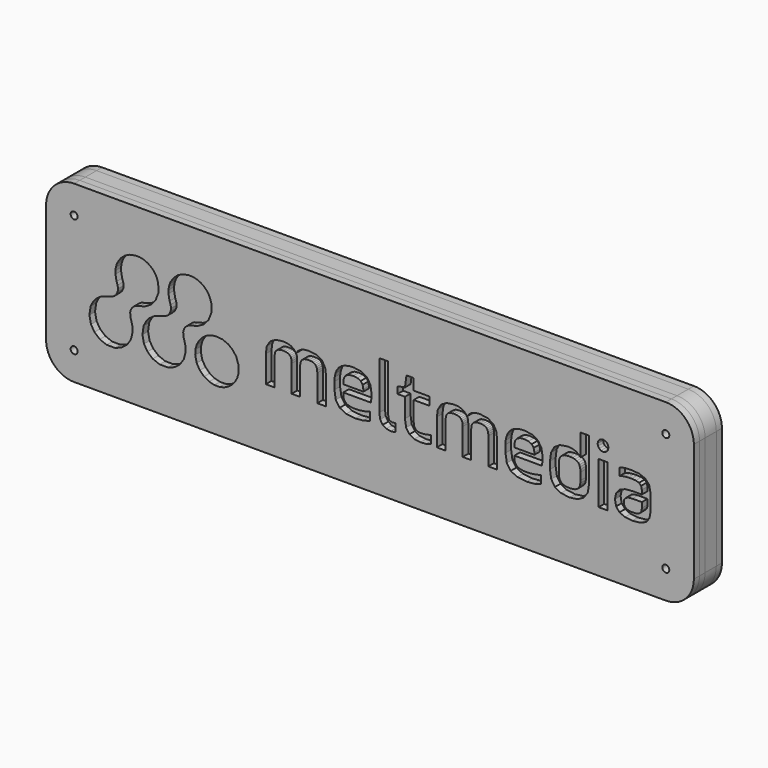
from build123d import *

# Parameters (mm, degrees)
F0_R     = 1.5875
F0_W     = 3.98907
F0_H     = 19.209766
F1_DEPTH = 3.175
F2_DEPTH = 3.175
F3_R     = 1.5875
F4_DEPTH = 6.35
F5_R     = 1.5875
F6_DEPTH = 3.175
F7_SIZE  = 3.17499
F9_DEPTH = 6.35


# Not quite as in the source:
# - a fillet or chamfer is up to 0.001 mm smaller than in the source, because OpenCascade refuses the exact size


with BuildPart() as f1:
    # F0 (on Front) → F1 (new body)
    with BuildSketch(Plane.XZ):
        with BuildLine():
            Line((133.9048122, 39.625524), (-133.9048122, 39.625524))
            ThreePointArc((-133.9048122, 39.625524), (-142.8850683211, 35.9057801211), (-146.6048122, 26.925524))
            Line((-146.6048122, 26.925524), (-146.6048122, -26.747978))
            ThreePointArc((-146.6048122, -26.747978), (-142.8850683211, -35.7282341211), (-133.9048122, -39.447978))
            Line((-133.9048122, -39.447978), (133.9048122, -39.447978))
            ThreePointArc((133.9048122, -39.447978), (142.8850683211, -35.7282341211), (146.6048122, -26.747978))
            Line((146.6048122, -26.747978), (146.6048122, 26.925524))
            ThreePointArc((146.6048122, 26.925524), (142.8850683211, 35.9057801211), (133.9048122, 39.625524))
        make_face()
        with Locations((-133.9048122, -26.747978)):
            Circle(F0_R, mode=Mode.SUBTRACT)
        Polygon((-70.4247258, -19.990562), (-72.7785438, -19.371818), (-75.0564158, -18.125948), (-77.0119618, -16.276828), (-78.4310598, -13.852906), (-79.0983178, -10.884662), (-79.0058618, -8.631428), (-78.4836378, -6.670294), (-77.6553438, -5.001768), (-76.6398518, -3.628898), (-75.4381778, -2.464816), (-73.9469438, -1.46431), (-72.1763098, -0.73787), (-70.0843658, -0.352044), (-66.8240218, -0.596138), (-64.0927598, -1.726184), (-61.9581438, -3.469132), (-60.4864678, -5.559806), (-59.5052658, -8.523732), (-59.4915498, -11.765026), (-60.0620338, -13.778484), (-61.0569518, -15.633446), (-62.4209318, -17.257776), (-64.0968238, -18.578068), (-66.0259538, -19.520662), (-68.1549818, -20.016724), align=None, mode=Mode.SUBTRACT)
        Polygon((-43.1728118, 0.021082), (-43.1728118, -12.099798), (-47.1618818, -12.099798), (-47.1618818, 0.021082), (-46.6907118, 3.205988), (-45.2505318, 5.56514), (-42.8007018, 7.031228), (-39.3003278, 7.534402), (-37.2718838, 7.344156), (-35.6417118, 6.788912), (-34.3889838, 5.901182), (-33.4908398, 4.706874), (-32.5672958, 5.901182), (-31.2983118, 6.788912), (-29.6734738, 7.344156), (-27.6823678, 7.534402), (-24.1075718, 7.042404), (-21.6793318, 5.594096), (-20.2973178, 3.237738), (-19.8591678, 0.021082), (-19.8591678, -12.099798), (-23.8472218, -12.099798), (-23.8472218, 0.021082), (-23.8843058, 0.885444), (-24.0057178, 1.64465), (-24.2343178, 2.295144), (-24.5883938, 2.835402), (-25.0900438, 3.259582), (-25.7595878, 3.566922), (-26.6168378, 3.754374), (-27.6823678, 3.81635), (-28.7626298, 3.754374), (-29.6335958, 3.566922), (-30.3158398, 3.259582), (-30.8284118, 2.835402), (-31.1934098, 2.295144), (-31.4291218, 1.64465), (-31.5558678, 0.885444), (-31.5932058, 0.021082), (-31.5932058, -12.099798), (-35.4651818, -12.099798), (-35.4651818, 0.021082), (-35.5012498, 0.885444), (-35.6183438, 1.64465), (-35.8416098, 2.295144), (-36.1931458, 2.835402), (-36.6920018, 3.259582), (-37.3615458, 3.566922), (-38.2241298, 3.754374), (-39.3003278, 3.81635), (-40.3795738, 3.754374), (-41.2462218, 3.566922), (-41.9213538, 3.259582), (-42.4273218, 2.835402), (-42.7854618, 2.295144), (-43.0143158, 1.64465), (-43.1367438, 0.885444), align=None, mode=Mode.SUBTRACT)
        Polygon((0.6655562, -2.151888), (0.3569462, -3.967988), (-12.0743218, -3.967988), (-12.0743218, -4.81965), (-11.9973598, -5.801106), (-11.7603778, -6.629146), (-11.3539778, -7.31139), (-10.7723178, -7.854188), (-10.0075238, -8.264906), (-9.0524838, -8.548878), (-7.8977998, -8.715248), (-6.5361058, -8.76935), (-4.7555658, -8.679688), (-2.9201618, -8.439912), (-1.2376658, -8.082788), (0.0851662, -7.647432), (0.0851662, -11.402568), (-3.0509718, -12.24026), (-6.5361058, -12.527026), (-10.7377738, -12.063984), (-13.7116058, -10.604754), (-15.4796998, -8.031988), (-16.0638998, -4.238244), (-16.0638998, -0.868934), (-15.9605218, 0.88265), (-15.6310838, 2.48666), (-15.0496778, 3.918204), (-14.1909038, 5.149088), (-13.0296158, 6.152134), (-11.5383818, 6.903212), (-9.6920558, 7.373112), (-7.4649838, 7.534402), (-3.9290498, 7.028688), (-1.3575538, 5.517134), (0.2121662, 3.010154), (0.7437882, -0.481584), align=None, mode=Mode.SUBTRACT)
        with Locations((133.9048122, -26.747978)):
            Circle(F0_R, mode=Mode.SUBTRACT)
        Polygon((12.4778262, 3.390646), (12.4778262, 6.48843), (15.8473902, 7.108444), (16.5060122, 12.142724), (19.7981062, 12.142724), (19.7981062, 7.108444), (26.8468602, 7.108444), (26.8468602, 3.390646), (19.7981062, 3.390646), (19.7981062, -5.40004), (20.0132442, -7.00405), (20.6248762, -8.04291), (21.5786462, -8.602472), (22.8189282, -8.770366), (24.1333782, -8.708644), (25.4135382, -8.537448), (26.5766042, -8.278622), (27.5440902, -7.956296), (27.5440902, -11.674094), (25.3845822, -12.28344), (22.8189282, -12.487148), (20.0295002, -12.130278), (17.8222402, -10.94232), (16.3693602, -8.745728), (15.8473902, -5.361178), (15.8473902, 3.390646), align=None, mode=Mode.SUBTRACT)
        Polygon((34.2438482, 0.021082), (34.2438482, -12.099798), (30.2547782, -12.099798), (30.2547782, 0.021082), (30.7259482, 3.205988), (32.1661282, 5.56514), (34.6162122, 7.031228), (38.1163322, 7.534402), (40.1447762, 7.344156), (41.7749482, 6.788912), (43.0276762, 5.901182), (43.9263282, 4.706874), (44.8496182, 5.901182), (46.1173322, 6.788912), (47.7419162, 7.344156), (49.7348002, 7.534402), (53.3090882, 7.042404), (55.7373282, 5.594096), (57.1195962, 3.237738), (57.5577462, 0.021082), (57.5577462, -12.099798), (53.5684222, -12.099798), (53.5684222, 0.021082), (53.5310842, 0.885444), (53.4099262, 1.64465), (53.1825962, 2.295144), (52.8269962, 2.835402), (52.3253462, 3.259582), (51.6570722, 3.566922), (50.7998222, 3.754374), (49.7348002, 3.81635), (48.6542842, 3.754374), (47.7833182, 3.566922), (47.1013282, 3.259582), (46.5887562, 2.835402), (46.2232502, 2.295144), (45.9875382, 1.64465), (45.8610462, 0.885444), (45.8239622, 0.021082), (45.8239622, -12.099798), (41.9499542, -12.099798), (41.9499542, 0.021082), (41.9154102, 0.885444), (41.7973002, 1.64465), (41.5740342, 2.295144), (41.2240222, 2.835402), (40.7251662, 3.259582), (40.0553682, 3.566922), (39.1927842, 3.754374), (38.1163322, 3.81635), (37.0373402, 3.754374), (36.1704382, 3.566922), (35.4953062, 3.259582), (34.9898462, 2.835402), (34.6311982, 2.295144), (34.4025982, 1.64465), (34.2799162, 0.885444), align=None, mode=Mode.SUBTRACT)
        Polygon((78.0822162, -2.151888), (77.7736062, -3.967988), (65.3423382, -3.967988), (65.3423382, -4.81965), (65.4195542, -5.801106), (65.6562822, -6.629146), (66.0631902, -7.31139), (66.6445962, -7.854188), (67.4093902, -8.264906), (68.3641762, -8.548878), (69.5193682, -8.715248), (70.8805542, -8.76935), (72.6610942, -8.679688), (74.4964982, -8.439912), (76.1792482, -8.082788), (77.5033502, -7.647432), (77.5033502, -11.402568), (74.3656882, -12.24026), (70.8805542, -12.527026), (66.6791402, -12.063984), (63.7050542, -10.604754), (61.9369602, -8.031988), (61.3527602, -4.238244), (61.3527602, -0.868934), (61.4561382, 0.88265), (61.7855762, 2.48666), (62.3669822, 3.918204), (63.2257562, 5.149088), (64.3872982, 6.152134), (65.8782782, 6.903212), (67.7251122, 7.373112), (69.9516762, 7.534402), (73.4881182, 7.028688), (76.0593602, 5.517134), (77.6288262, 3.010154), (78.1609562, -0.481584), align=None, mode=Mode.SUBTRACT)
        with Locations((105.4838632, -2.496439)):
            Rectangle(F0_W, F0_H, mode=Mode.SUBTRACT)
        Polygon((126.9960122, 1.182878), (126.9960122, -6.330188), (126.5134122, -9.09574), (125.0198922, -11.026394), (122.4544922, -12.15771), (118.7486322, -12.527026), (115.3958322, -12.171426), (112.9294922, -11.084306), (111.4054922, -9.22655), (110.8873322, -6.563106), (111.4385122, -3.817874), (113.0209322, -2.011172), (115.5101322, -1.017778), (118.7867322, -0.714756), (123.0463122, -0.714756), (123.0463122, 1.182878), (122.7186522, 2.657602), (121.7915522, 3.556), (120.3488322, 4.005072), (118.4768522, 4.126484), (116.8258522, 4.0767), (115.3323322, 3.933444), (114.0369322, 3.70205), (112.9777522, 3.390646), (112.9777522, 6.87578), (115.3475722, 7.380224), (118.2431722, 7.534402), (121.8169522, 7.222744), (124.5804722, 6.174232), (126.3635522, 4.21894), align=None, mode=Mode.SUBTRACT)
        Polygon((-108.2463418, -2.313178), (-108.5386958, -3.510534), (-108.3690238, -5.424678), (-107.8950598, -7.140194), (-107.5064398, -8.887968), (-107.4276998, -10.945368), (-108.2450718, -14.208506), (-110.0060538, -16.862298), (-112.4962698, -18.78076), (-115.5018518, -19.839178), (-119.1907954, -19.839178), (-122.2982822, -18.631916), (-124.7002078, -16.56461), (-126.2711724, -13.98651), (-126.9960122, -10.529062), (-126.44755, -6.846824), (-125.4043974, -4.764532), (-123.9381316, -2.996438), (-122.07367, -1.617218), (-119.8343552, -0.702056), (-118.1572694, -0.294132), (-116.5574758, 0.236474), (-115.5859258, 0.853694), (-114.7797298, 1.738376), (-114.2338838, 2.865628), (-114.0383038, 4.211828), (-114.2724918, 5.567934), (-114.6847338, 6.848094), (-115.2097518, 9.59866), (-115.2122918, 11.056874), (-115.0098538, 12.452604), (-114.6296158, 13.753338), (-114.0974858, 14.924532), (-112.8008158, 16.7767), (-110.9956378, 18.378424), (-108.7535798, 19.476466), (-105.9628818, 20.016724), (-103.9829518, 19.937984), (-102.1417058, 19.472402), (-100.5143278, 18.722594), (-99.1734618, 17.793716), (-98.0434158, 16.705072), (-97.0871058, 15.432024), (-96.3403458, 13.935456), (-95.8371718, 12.17295), (-95.8125338, 8.277352), (-97.0952338, 5.019294), (-99.3151938, 2.543302), (-102.1003038, 0.994156), (-104.1013158, 0.518922), (-106.0802298, -0.059944), (-106.9402738, -0.589026), (-107.6883038, -1.340104), align=None, mode=Mode.SUBTRACT)
        Polygon((-84.2476598, -2.313178), (-84.5412838, -3.510534), (-84.3718658, -5.424678), (-83.8963778, -7.140194), (-83.5092818, -8.887968), (-83.4292718, -10.945368), (-84.2476598, -14.208506), (-86.0091498, -16.862298), (-88.5003818, -18.78076), (-91.5062178, -19.839178), (-95.1950598, -19.839178), (-98.3024958, -18.631916), (-100.7045738, -16.56461), (-102.2753098, -13.98651), (-102.9989558, -10.529062), (-102.4503158, -6.846824), (-101.4071378, -4.764532), (-99.9410498, -2.996438), (-98.0766898, -1.617218), (-95.8371718, -0.702056), (-94.1600098, -0.294132), (-92.5587938, 0.236474), (-91.5887678, 0.853694), (-90.7840958, 1.738376), (-90.2382498, 2.865628), (-90.0439398, 4.211828), (-90.2753338, 5.567934), (-90.6860518, 6.848094), (-91.2125938, 9.59866), (-91.2151338, 11.056874), (-91.0126958, 12.452604), (-90.6322038, 13.753338), (-90.1003278, 14.924532), (-88.8049278, 16.7767), (-86.9997498, 18.378424), (-84.7564218, 19.476466), (-81.9631838, 20.016724), (-79.9855398, 19.937984), (-78.1448018, 19.472402), (-76.5169158, 18.722594), (-75.1750338, 17.793716), (-74.0460038, 16.705072), (-73.0902018, 15.432024), (-72.3429338, 13.935456), (-71.8402678, 12.17295), (-71.8151218, 8.277352), (-73.0980758, 5.019294), (-75.3167658, 2.543302), (-78.1031458, 0.994156), (-80.1054278, 0.518922), (-82.0818018, -0.059944), (-82.9428618, -0.589026), (-83.6896218, -1.340104), align=None, mode=Mode.SUBTRACT)
        with Locations((-133.9048122, 26.925524)):
            Circle(F0_R, mode=Mode.SUBTRACT)
        Polygon((4.2289222, -6.678676), (4.2289222, 15.00886), (8.2200242, 15.00886), (8.2200242, -5.904484), (8.3399122, -7.24789), (8.6927182, -8.09117), (9.2644722, -8.52805), (10.0389182, -8.653272), (10.7884722, -8.609076), (11.5105942, -8.421878), (11.5105942, -12.061444), (10.5763822, -12.321794), (9.3802962, -12.409932), (7.3655682, -12.097004), (5.7295542, -11.098022), (4.6299882, -9.3218), align=None, mode=Mode.SUBTRACT)
        Polygon((99.1911402, 15.00886), (99.1911402, -4.238244), (98.5723962, -7.917688), (96.8083662, -10.501376), (94.0260502, -12.025376), (90.3605762, -12.525756), (86.4911402, -12.025376), (83.7184762, -10.501376), (82.0481722, -7.917688), (81.4914042, -4.238244), (81.4914042, -0.907288), (81.9656222, 2.65049), (83.4317102, 5.303266), (85.9524062, 6.962394), (89.5858762, 7.534402), (91.5746962, 7.359396), (93.1525442, 6.856222), (94.3610762, 6.063996), (95.2401702, 5.016754), (95.2401702, 15.00886), align=None, mode=Mode.SUBTRACT)
        Polygon((104.5434282, 15.28318), (105.5035482, 15.473172), (106.4560482, 15.277338), (107.2304942, 14.748256), (107.7514482, 13.971016), (107.9432182, 13.03401), (107.7514482, 12.082018), (107.2304942, 11.306302), (106.4560482, 10.785094), (105.5035482, 10.593578), (104.5434282, 10.785094), (103.7550122, 11.306302), (103.2205962, 12.082018), (103.0247622, 13.03401), (103.2205962, 13.98778), (103.7550122, 14.762226), align=None, mode=Mode.SUBTRACT)
        with Locations((133.9048122, 26.925524)):
            Circle(F0_R, mode=Mode.SUBTRACT)
    extrude(amount=F1_DEPTH)


with BuildPart() as f1b:
    # F0 (on Front) → F1, piece 2 (new body)
    with BuildSketch(Plane.XZ):
        Polygon((-12.0743218, 0.254254), (-12.0743218, -0.714756), (-3.0126178, -0.714756), (-3.0126178, 0.254254), (-3.3184338, 1.964182), (-4.2087038, 3.159252), (-5.6432958, 3.860546), (-7.5820778, 4.087876), (-9.5099378, 3.860546), (-10.9183678, 3.159252), (-11.7822218, 1.964182), align=None)
    extrude(amount=F1_DEPTH)


with BuildPart() as f1c:
    # F0 (on Front) → F1, piece 3 (new body)
    with BuildSketch(Plane.XZ):
        Polygon((65.3423382, 0.254254), (65.3423382, -0.714756), (74.4042962, -0.714756), (74.4042962, 0.254254), (74.0982262, 1.964182), (73.2082102, 3.159252), (71.7736182, 3.860546), (69.8345822, 4.087876), (67.9067222, 3.860546), (66.4985462, 3.159252), (65.6344382, 1.964182), align=None)
    extrude(amount=F1_DEPTH)


with BuildPart() as f1d:
    # F0 (on Front) → F1, piece 4 (new body)
    with BuildSketch(Plane.XZ):
        Polygon((85.4809822, -0.830326), (85.4809822, -4.161028), (85.5236542, -5.226304), (85.6697042, -6.154928), (85.9496122, -6.946138), (86.3905562, -7.597648), (87.0186982, -8.107934), (87.8647722, -8.474456), (88.9562102, -8.696198), (90.3219682, -8.770366), (91.6778202, -8.696198), (92.7723062, -8.474456), (93.6305722, -8.107934), (94.2754782, -7.597648), (94.7344562, -6.946138), (95.0321442, -6.154928), (95.1919102, -5.226304), (95.2401702, -4.161028), (95.2401702, -0.830326), (95.1919102, 0.237744), (95.0321442, 1.170432), (94.7344562, 1.9685), (94.2754782, 2.625852), (93.6305722, 3.144012), (92.7723062, 3.516122), (91.6778202, 3.741928), (90.3219682, 3.81635), (88.9785622, 3.741928), (87.8980462, 3.516122), (87.0534962, 3.144012), (86.4195122, 2.625852), (85.9699322, 1.9685), (85.6806262, 1.170432), (85.5264482, 0.237744), align=None)
    extrude(amount=F1_DEPTH)


with BuildPart() as f1e:
    # F0 (on Front) → F1, piece 5 (new body)
    with BuildSketch(Plane.XZ):
        Polygon((123.0463122, -6.137148), (123.0463122, -3.73507), (118.7867322, -3.73507), (117.0646122, -3.886962), (115.8428722, -4.369054), (115.1138922, -5.22224), (114.8751322, -6.48589), (115.1875522, -7.866634), (116.0308322, -8.678418), (117.2424122, -9.06145), (118.6698922, -9.157716), (119.5817522, -9.135872), (120.4148722, -9.055862), (121.1590922, -8.896096), (121.8017122, -8.634222), (122.3249522, -8.249666), (122.7161122, -7.71906), (122.9599522, -7.021576), align=None)
    extrude(amount=F1_DEPTH)


with BuildPart() as f2:
    # F0 (on Front) → F2 (new body)
    with BuildSketch(Plane.XZ):
        with BuildLine():
            Line((133.9048122, 39.625524), (-133.9048122, 39.625524))
            ThreePointArc((-133.9048122, 39.625524), (-142.8850683211, 35.9057801211), (-146.6048122, 26.925524))
            Line((-146.6048122, 26.925524), (-146.6048122, -26.747978))
            ThreePointArc((-146.6048122, -26.747978), (-142.8850683211, -35.7282341211), (-133.9048122, -39.447978))
            Line((-133.9048122, -39.447978), (133.9048122, -39.447978))
            ThreePointArc((133.9048122, -39.447978), (142.8850683211, -35.7282341211), (146.6048122, -26.747978))
            Line((146.6048122, -26.747978), (146.6048122, 26.925524))
            ThreePointArc((146.6048122, 26.925524), (142.8850683211, 35.9057801211), (133.9048122, 39.625524))
        make_face()
        with Locations((-133.9048122, -26.747978)):
            Circle(F0_R, mode=Mode.SUBTRACT)
        Polygon((-70.4247258, -19.990562), (-72.7785438, -19.371818), (-75.0564158, -18.125948), (-77.0119618, -16.276828), (-78.4310598, -13.852906), (-79.0983178, -10.884662), (-79.0058618, -8.631428), (-78.4836378, -6.670294), (-77.6553438, -5.001768), (-76.6398518, -3.628898), (-75.4381778, -2.464816), (-73.9469438, -1.46431), (-72.1763098, -0.73787), (-70.0843658, -0.352044), (-66.8240218, -0.596138), (-64.0927598, -1.726184), (-61.9581438, -3.469132), (-60.4864678, -5.559806), (-59.5052658, -8.523732), (-59.4915498, -11.765026), (-60.0620338, -13.778484), (-61.0569518, -15.633446), (-62.4209318, -17.257776), (-64.0968238, -18.578068), (-66.0259538, -19.520662), (-68.1549818, -20.016724), align=None, mode=Mode.SUBTRACT)
        Polygon((-43.1728118, 0.021082), (-43.1728118, -12.099798), (-47.1618818, -12.099798), (-47.1618818, 0.021082), (-46.6907118, 3.205988), (-45.2505318, 5.56514), (-42.8007018, 7.031228), (-39.3003278, 7.534402), (-37.2718838, 7.344156), (-35.6417118, 6.788912), (-34.3889838, 5.901182), (-33.4908398, 4.706874), (-32.5672958, 5.901182), (-31.2983118, 6.788912), (-29.6734738, 7.344156), (-27.6823678, 7.534402), (-24.1075718, 7.042404), (-21.6793318, 5.594096), (-20.2973178, 3.237738), (-19.8591678, 0.021082), (-19.8591678, -12.099798), (-23.8472218, -12.099798), (-23.8472218, 0.021082), (-23.8843058, 0.885444), (-24.0057178, 1.64465), (-24.2343178, 2.295144), (-24.5883938, 2.835402), (-25.0900438, 3.259582), (-25.7595878, 3.566922), (-26.6168378, 3.754374), (-27.6823678, 3.81635), (-28.7626298, 3.754374), (-29.6335958, 3.566922), (-30.3158398, 3.259582), (-30.8284118, 2.835402), (-31.1934098, 2.295144), (-31.4291218, 1.64465), (-31.5558678, 0.885444), (-31.5932058, 0.021082), (-31.5932058, -12.099798), (-35.4651818, -12.099798), (-35.4651818, 0.021082), (-35.5012498, 0.885444), (-35.6183438, 1.64465), (-35.8416098, 2.295144), (-36.1931458, 2.835402), (-36.6920018, 3.259582), (-37.3615458, 3.566922), (-38.2241298, 3.754374), (-39.3003278, 3.81635), (-40.3795738, 3.754374), (-41.2462218, 3.566922), (-41.9213538, 3.259582), (-42.4273218, 2.835402), (-42.7854618, 2.295144), (-43.0143158, 1.64465), (-43.1367438, 0.885444), align=None, mode=Mode.SUBTRACT)
        Polygon((0.6655562, -2.151888), (0.3569462, -3.967988), (-12.0743218, -3.967988), (-12.0743218, -4.81965), (-11.9973598, -5.801106), (-11.7603778, -6.629146), (-11.3539778, -7.31139), (-10.7723178, -7.854188), (-10.0075238, -8.264906), (-9.0524838, -8.548878), (-7.8977998, -8.715248), (-6.5361058, -8.76935), (-4.7555658, -8.679688), (-2.9201618, -8.439912), (-1.2376658, -8.082788), (0.0851662, -7.647432), (0.0851662, -11.402568), (-3.0509718, -12.24026), (-6.5361058, -12.527026), (-10.7377738, -12.063984), (-13.7116058, -10.604754), (-15.4796998, -8.031988), (-16.0638998, -4.238244), (-16.0638998, -0.868934), (-15.9605218, 0.88265), (-15.6310838, 2.48666), (-15.0496778, 3.918204), (-14.1909038, 5.149088), (-13.0296158, 6.152134), (-11.5383818, 6.903212), (-9.6920558, 7.373112), (-7.4649838, 7.534402), (-3.9290498, 7.028688), (-1.3575538, 5.517134), (0.2121662, 3.010154), (0.7437882, -0.481584), align=None, mode=Mode.SUBTRACT)
        with Locations((133.9048122, -26.747978)):
            Circle(F0_R, mode=Mode.SUBTRACT)
        Polygon((12.4778262, 3.390646), (12.4778262, 6.48843), (15.8473902, 7.108444), (16.5060122, 12.142724), (19.7981062, 12.142724), (19.7981062, 7.108444), (26.8468602, 7.108444), (26.8468602, 3.390646), (19.7981062, 3.390646), (19.7981062, -5.40004), (20.0132442, -7.00405), (20.6248762, -8.04291), (21.5786462, -8.602472), (22.8189282, -8.770366), (24.1333782, -8.708644), (25.4135382, -8.537448), (26.5766042, -8.278622), (27.5440902, -7.956296), (27.5440902, -11.674094), (25.3845822, -12.28344), (22.8189282, -12.487148), (20.0295002, -12.130278), (17.8222402, -10.94232), (16.3693602, -8.745728), (15.8473902, -5.361178), (15.8473902, 3.390646), align=None, mode=Mode.SUBTRACT)
        Polygon((34.2438482, 0.021082), (34.2438482, -12.099798), (30.2547782, -12.099798), (30.2547782, 0.021082), (30.7259482, 3.205988), (32.1661282, 5.56514), (34.6162122, 7.031228), (38.1163322, 7.534402), (40.1447762, 7.344156), (41.7749482, 6.788912), (43.0276762, 5.901182), (43.9263282, 4.706874), (44.8496182, 5.901182), (46.1173322, 6.788912), (47.7419162, 7.344156), (49.7348002, 7.534402), (53.3090882, 7.042404), (55.7373282, 5.594096), (57.1195962, 3.237738), (57.5577462, 0.021082), (57.5577462, -12.099798), (53.5684222, -12.099798), (53.5684222, 0.021082), (53.5310842, 0.885444), (53.4099262, 1.64465), (53.1825962, 2.295144), (52.8269962, 2.835402), (52.3253462, 3.259582), (51.6570722, 3.566922), (50.7998222, 3.754374), (49.7348002, 3.81635), (48.6542842, 3.754374), (47.7833182, 3.566922), (47.1013282, 3.259582), (46.5887562, 2.835402), (46.2232502, 2.295144), (45.9875382, 1.64465), (45.8610462, 0.885444), (45.8239622, 0.021082), (45.8239622, -12.099798), (41.9499542, -12.099798), (41.9499542, 0.021082), (41.9154102, 0.885444), (41.7973002, 1.64465), (41.5740342, 2.295144), (41.2240222, 2.835402), (40.7251662, 3.259582), (40.0553682, 3.566922), (39.1927842, 3.754374), (38.1163322, 3.81635), (37.0373402, 3.754374), (36.1704382, 3.566922), (35.4953062, 3.259582), (34.9898462, 2.835402), (34.6311982, 2.295144), (34.4025982, 1.64465), (34.2799162, 0.885444), align=None, mode=Mode.SUBTRACT)
        Polygon((78.0822162, -2.151888), (77.7736062, -3.967988), (65.3423382, -3.967988), (65.3423382, -4.81965), (65.4195542, -5.801106), (65.6562822, -6.629146), (66.0631902, -7.31139), (66.6445962, -7.854188), (67.4093902, -8.264906), (68.3641762, -8.548878), (69.5193682, -8.715248), (70.8805542, -8.76935), (72.6610942, -8.679688), (74.4964982, -8.439912), (76.1792482, -8.082788), (77.5033502, -7.647432), (77.5033502, -11.402568), (74.3656882, -12.24026), (70.8805542, -12.527026), (66.6791402, -12.063984), (63.7050542, -10.604754), (61.9369602, -8.031988), (61.3527602, -4.238244), (61.3527602, -0.868934), (61.4561382, 0.88265), (61.7855762, 2.48666), (62.3669822, 3.918204), (63.2257562, 5.149088), (64.3872982, 6.152134), (65.8782782, 6.903212), (67.7251122, 7.373112), (69.9516762, 7.534402), (73.4881182, 7.028688), (76.0593602, 5.517134), (77.6288262, 3.010154), (78.1609562, -0.481584), align=None, mode=Mode.SUBTRACT)
        with Locations((105.4838632, -2.496439)):
            Rectangle(F0_W, F0_H, mode=Mode.SUBTRACT)
        Polygon((126.9960122, 1.182878), (126.9960122, -6.330188), (126.5134122, -9.09574), (125.0198922, -11.026394), (122.4544922, -12.15771), (118.7486322, -12.527026), (115.3958322, -12.171426), (112.9294922, -11.084306), (111.4054922, -9.22655), (110.8873322, -6.563106), (111.4385122, -3.817874), (113.0209322, -2.011172), (115.5101322, -1.017778), (118.7867322, -0.714756), (123.0463122, -0.714756), (123.0463122, 1.182878), (122.7186522, 2.657602), (121.7915522, 3.556), (120.3488322, 4.005072), (118.4768522, 4.126484), (116.8258522, 4.0767), (115.3323322, 3.933444), (114.0369322, 3.70205), (112.9777522, 3.390646), (112.9777522, 6.87578), (115.3475722, 7.380224), (118.2431722, 7.534402), (121.8169522, 7.222744), (124.5804722, 6.174232), (126.3635522, 4.21894), align=None, mode=Mode.SUBTRACT)
        Polygon((-108.2463418, -2.313178), (-108.5386958, -3.510534), (-108.3690238, -5.424678), (-107.8950598, -7.140194), (-107.5064398, -8.887968), (-107.4276998, -10.945368), (-108.2450718, -14.208506), (-110.0060538, -16.862298), (-112.4962698, -18.78076), (-115.5018518, -19.839178), (-119.1907954, -19.839178), (-122.2982822, -18.631916), (-124.7002078, -16.56461), (-126.2711724, -13.98651), (-126.9960122, -10.529062), (-126.44755, -6.846824), (-125.4043974, -4.764532), (-123.9381316, -2.996438), (-122.07367, -1.617218), (-119.8343552, -0.702056), (-118.1572694, -0.294132), (-116.5574758, 0.236474), (-115.5859258, 0.853694), (-114.7797298, 1.738376), (-114.2338838, 2.865628), (-114.0383038, 4.211828), (-114.2724918, 5.567934), (-114.6847338, 6.848094), (-115.2097518, 9.59866), (-115.2122918, 11.056874), (-115.0098538, 12.452604), (-114.6296158, 13.753338), (-114.0974858, 14.924532), (-112.8008158, 16.7767), (-110.9956378, 18.378424), (-108.7535798, 19.476466), (-105.9628818, 20.016724), (-103.9829518, 19.937984), (-102.1417058, 19.472402), (-100.5143278, 18.722594), (-99.1734618, 17.793716), (-98.0434158, 16.705072), (-97.0871058, 15.432024), (-96.3403458, 13.935456), (-95.8371718, 12.17295), (-95.8125338, 8.277352), (-97.0952338, 5.019294), (-99.3151938, 2.543302), (-102.1003038, 0.994156), (-104.1013158, 0.518922), (-106.0802298, -0.059944), (-106.9402738, -0.589026), (-107.6883038, -1.340104), align=None, mode=Mode.SUBTRACT)
        Polygon((-84.2476598, -2.313178), (-84.5412838, -3.510534), (-84.3718658, -5.424678), (-83.8963778, -7.140194), (-83.5092818, -8.887968), (-83.4292718, -10.945368), (-84.2476598, -14.208506), (-86.0091498, -16.862298), (-88.5003818, -18.78076), (-91.5062178, -19.839178), (-95.1950598, -19.839178), (-98.3024958, -18.631916), (-100.7045738, -16.56461), (-102.2753098, -13.98651), (-102.9989558, -10.529062), (-102.4503158, -6.846824), (-101.4071378, -4.764532), (-99.9410498, -2.996438), (-98.0766898, -1.617218), (-95.8371718, -0.702056), (-94.1600098, -0.294132), (-92.5587938, 0.236474), (-91.5887678, 0.853694), (-90.7840958, 1.738376), (-90.2382498, 2.865628), (-90.0439398, 4.211828), (-90.2753338, 5.567934), (-90.6860518, 6.848094), (-91.2125938, 9.59866), (-91.2151338, 11.056874), (-91.0126958, 12.452604), (-90.6322038, 13.753338), (-90.1003278, 14.924532), (-88.8049278, 16.7767), (-86.9997498, 18.378424), (-84.7564218, 19.476466), (-81.9631838, 20.016724), (-79.9855398, 19.937984), (-78.1448018, 19.472402), (-76.5169158, 18.722594), (-75.1750338, 17.793716), (-74.0460038, 16.705072), (-73.0902018, 15.432024), (-72.3429338, 13.935456), (-71.8402678, 12.17295), (-71.8151218, 8.277352), (-73.0980758, 5.019294), (-75.3167658, 2.543302), (-78.1031458, 0.994156), (-80.1054278, 0.518922), (-82.0818018, -0.059944), (-82.9428618, -0.589026), (-83.6896218, -1.340104), align=None, mode=Mode.SUBTRACT)
        with Locations((-133.9048122, 26.925524)):
            Circle(F0_R, mode=Mode.SUBTRACT)
        Polygon((4.2289222, -6.678676), (4.2289222, 15.00886), (8.2200242, 15.00886), (8.2200242, -5.904484), (8.3399122, -7.24789), (8.6927182, -8.09117), (9.2644722, -8.52805), (10.0389182, -8.653272), (10.7884722, -8.609076), (11.5105942, -8.421878), (11.5105942, -12.061444), (10.5763822, -12.321794), (9.3802962, -12.409932), (7.3655682, -12.097004), (5.7295542, -11.098022), (4.6299882, -9.3218), align=None, mode=Mode.SUBTRACT)
        Polygon((99.1911402, 15.00886), (99.1911402, -4.238244), (98.5723962, -7.917688), (96.8083662, -10.501376), (94.0260502, -12.025376), (90.3605762, -12.525756), (86.4911402, -12.025376), (83.7184762, -10.501376), (82.0481722, -7.917688), (81.4914042, -4.238244), (81.4914042, -0.907288), (81.9656222, 2.65049), (83.4317102, 5.303266), (85.9524062, 6.962394), (89.5858762, 7.534402), (91.5746962, 7.359396), (93.1525442, 6.856222), (94.3610762, 6.063996), (95.2401702, 5.016754), (95.2401702, 15.00886), align=None, mode=Mode.SUBTRACT)
        Polygon((104.5434282, 15.28318), (105.5035482, 15.473172), (106.4560482, 15.277338), (107.2304942, 14.748256), (107.7514482, 13.971016), (107.9432182, 13.03401), (107.7514482, 12.082018), (107.2304942, 11.306302), (106.4560482, 10.785094), (105.5035482, 10.593578), (104.5434282, 10.785094), (103.7550122, 11.306302), (103.2205962, 12.082018), (103.0247622, 13.03401), (103.2205962, 13.98778), (103.7550122, 14.762226), align=None, mode=Mode.SUBTRACT)
        with Locations((133.9048122, 26.925524)):
            Circle(F0_R, mode=Mode.SUBTRACT)
        Polygon((-84.3718658, -5.424678), (-84.5412838, -3.510534), (-84.2476598, -2.313178), (-83.6896218, -1.340104), (-82.9428618, -0.589026), (-82.0818018, -0.059944), (-80.1054278, 0.518922), (-78.1031458, 0.994156), (-75.3167658, 2.543302), (-73.0980758, 5.019294), (-71.8151218, 8.277352), (-71.8402678, 12.17295), (-72.3429338, 13.935456), (-73.0902018, 15.432024), (-74.0460038, 16.705072), (-75.1750338, 17.793716), (-76.5169158, 18.722594), (-78.1448018, 19.472402), (-79.9855398, 19.937984), (-81.9631838, 20.016724), (-84.7564218, 19.476466), (-86.9997498, 18.378424), (-88.8049278, 16.7767), (-90.1003278, 14.924532), (-90.6322038, 13.753338), (-91.0126958, 12.452604), (-91.2151338, 11.056874), (-91.2125938, 9.59866), (-90.6860518, 6.848094), (-90.2753338, 5.567934), (-90.0439398, 4.211828), (-90.2382498, 2.865628), (-90.7840958, 1.738376), (-91.5887678, 0.853694), (-92.5587938, 0.236474), (-94.1600098, -0.294132), (-95.8371718, -0.702056), (-98.0766898, -1.617218), (-99.9410498, -2.996438), (-101.4071378, -4.764532), (-102.4503158, -6.846824), (-102.9989558, -10.529062), (-102.2753098, -13.98651), (-100.7045738, -16.56461), (-98.3024958, -18.631916), (-95.1950598, -19.839178), (-91.5062178, -19.839178), (-88.5003818, -18.78076), (-86.0091498, -16.862298), (-84.2476598, -14.208506), (-83.4292718, -10.945368), (-83.5092818, -8.887968), (-83.8963778, -7.140194), align=None)
        Polygon((-108.3690238, -5.424678), (-108.5386958, -3.510534), (-108.2463418, -2.313178), (-107.6883038, -1.340104), (-106.9402738, -0.589026), (-106.0802298, -0.059944), (-104.1013158, 0.518922), (-102.1003038, 0.994156), (-99.3151938, 2.543302), (-97.0952338, 5.019294), (-95.8125338, 8.277352), (-95.8371718, 12.17295), (-96.3403458, 13.935456), (-97.0871058, 15.432024), (-98.0434158, 16.705072), (-99.1734618, 17.793716), (-100.5143278, 18.722594), (-102.1417058, 19.472402), (-103.9829518, 19.937984), (-105.9628818, 20.016724), (-108.7535798, 19.476466), (-110.9956378, 18.378424), (-112.8008158, 16.7767), (-114.0974858, 14.924532), (-114.6296158, 13.753338), (-115.0098538, 12.452604), (-115.2122918, 11.056874), (-115.2097518, 9.59866), (-114.6847338, 6.848094), (-114.2724918, 5.567934), (-114.0383038, 4.211828), (-114.2338838, 2.865628), (-114.7797298, 1.738376), (-115.5859258, 0.853694), (-116.5574758, 0.236474), (-118.1572694, -0.294132), (-119.8343552, -0.702056), (-122.07367, -1.617218), (-123.9381316, -2.996438), (-125.4043974, -4.764532), (-126.44755, -6.846824), (-126.9960122, -10.529062), (-126.2711724, -13.98651), (-124.7002078, -16.56461), (-122.2982822, -18.631916), (-119.1907954, -19.839178), (-115.5018518, -19.839178), (-112.4962698, -18.78076), (-110.0060538, -16.862298), (-108.2450718, -14.208506), (-107.4276998, -10.945368), (-107.5064398, -8.887968), (-107.8950598, -7.140194), align=None)
        Polygon((98.5723962, -7.917688), (99.1911402, -4.238244), (99.1911402, 15.00886), (95.2401702, 15.00886), (95.2401702, 5.016754), (94.3610762, 6.063996), (93.1525442, 6.856222), (91.5746962, 7.359396), (89.5858762, 7.534402), (85.9524062, 6.962394), (83.4317102, 5.303266), (81.9656222, 2.65049), (81.4914042, -0.907288), (81.4914042, -4.238244), (82.0481722, -7.917688), (83.7184762, -10.501376), (86.4911402, -12.025376), (90.3605762, -12.525756), (94.0260502, -12.025376), (96.8083662, -10.501376), align=None)
        Polygon((85.5236542, -5.226304), (85.4809822, -4.161028), (85.4809822, -0.830326), (85.5264482, 0.237744), (85.6806262, 1.170432), (85.9699322, 1.9685), (86.4195122, 2.625852), (87.0534962, 3.144012), (87.8980462, 3.516122), (88.9785622, 3.741928), (90.3219682, 3.81635), (91.6778202, 3.741928), (92.7723062, 3.516122), (93.6305722, 3.144012), (94.2754782, 2.625852), (94.7344562, 1.9685), (95.0321442, 1.170432), (95.1919102, 0.237744), (95.2401702, -0.830326), (95.2401702, -4.161028), (95.1919102, -5.226304), (95.0321442, -6.154928), (94.7344562, -6.946138), (94.2754782, -7.597648), (93.6305722, -8.107934), (92.7723062, -8.474456), (91.6778202, -8.696198), (90.3219682, -8.770366), (88.9562102, -8.696198), (87.8647722, -8.474456), (87.0186982, -8.107934), (86.3905562, -7.597648), (85.9496122, -6.946138), (85.6697042, -6.154928), align=None, mode=Mode.SUBTRACT)
        Polygon((-75.0564158, -18.125948), (-72.7785438, -19.371818), (-70.4247258, -19.990562), (-68.1549818, -20.016724), (-66.0259538, -19.520662), (-64.0968238, -18.578068), (-62.4209318, -17.257776), (-61.0569518, -15.633446), (-60.0620338, -13.778484), (-59.4915498, -11.765026), (-59.5052658, -8.523732), (-60.4864678, -5.559806), (-61.9581438, -3.469132), (-64.0927598, -1.726184), (-66.8240218, -0.596138), (-70.0843658, -0.352044), (-72.1763098, -0.73787), (-73.9469438, -1.46431), (-75.4381778, -2.464816), (-76.6398518, -3.628898), (-77.6553438, -5.001768), (-78.4836378, -6.670294), (-79.0058618, -8.631428), (-79.0983178, -10.884662), (-78.4310598, -13.852906), (-77.0119618, -16.276828), align=None)
        Polygon((30.2547782, -12.099798), (34.2438482, -12.099798), (34.2438482, 0.021082), (34.2799162, 0.885444), (34.4025982, 1.64465), (34.6311982, 2.295144), (34.9898462, 2.835402), (35.4953062, 3.259582), (36.1704382, 3.566922), (37.0373402, 3.754374), (38.1163322, 3.81635), (39.1927842, 3.754374), (40.0553682, 3.566922), (40.7251662, 3.259582), (41.2240222, 2.835402), (41.5740342, 2.295144), (41.7973002, 1.64465), (41.9154102, 0.885444), (41.9499542, 0.021082), (41.9499542, -12.099798), (45.8239622, -12.099798), (45.8239622, 0.021082), (45.8610462, 0.885444), (45.9875382, 1.64465), (46.2232502, 2.295144), (46.5887562, 2.835402), (47.1013282, 3.259582), (47.7833182, 3.566922), (48.6542842, 3.754374), (49.7348002, 3.81635), (50.7998222, 3.754374), (51.6570722, 3.566922), (52.3253462, 3.259582), (52.8269962, 2.835402), (53.1825962, 2.295144), (53.4099262, 1.64465), (53.5310842, 0.885444), (53.5684222, 0.021082), (53.5684222, -12.099798), (57.5577462, -12.099798), (57.5577462, 0.021082), (57.1195962, 3.237738), (55.7373282, 5.594096), (53.3090882, 7.042404), (49.7348002, 7.534402), (47.7419162, 7.344156), (46.1173322, 6.788912), (44.8496182, 5.901182), (43.9263282, 4.706874), (43.0276762, 5.901182), (41.7749482, 6.788912), (40.1447762, 7.344156), (38.1163322, 7.534402), (34.6162122, 7.031228), (32.1661282, 5.56514), (30.7259482, 3.205988), (30.2547782, 0.021082), align=None)
        Polygon((-47.1618818, -12.099798), (-43.1728118, -12.099798), (-43.1728118, 0.021082), (-43.1367438, 0.885444), (-43.0143158, 1.64465), (-42.7854618, 2.295144), (-42.4273218, 2.835402), (-41.9213538, 3.259582), (-41.2462218, 3.566922), (-40.3795738, 3.754374), (-39.3003278, 3.81635), (-38.2241298, 3.754374), (-37.3615458, 3.566922), (-36.6920018, 3.259582), (-36.1931458, 2.835402), (-35.8416098, 2.295144), (-35.6183438, 1.64465), (-35.5012498, 0.885444), (-35.4651818, 0.021082), (-35.4651818, -12.099798), (-31.5932058, -12.099798), (-31.5932058, 0.021082), (-31.5558678, 0.885444), (-31.4291218, 1.64465), (-31.1934098, 2.295144), (-30.8284118, 2.835402), (-30.3158398, 3.259582), (-29.6335958, 3.566922), (-28.7626298, 3.754374), (-27.6823678, 3.81635), (-26.6168378, 3.754374), (-25.7595878, 3.566922), (-25.0900438, 3.259582), (-24.5883938, 2.835402), (-24.2343178, 2.295144), (-24.0057178, 1.64465), (-23.8843058, 0.885444), (-23.8472218, 0.021082), (-23.8472218, -12.099798), (-19.8591678, -12.099798), (-19.8591678, 0.021082), (-20.2973178, 3.237738), (-21.6793318, 5.594096), (-24.1075718, 7.042404), (-27.6823678, 7.534402), (-29.6734738, 7.344156), (-31.2983118, 6.788912), (-32.5672958, 5.901182), (-33.4908398, 4.706874), (-34.3889838, 5.901182), (-35.6417118, 6.788912), (-37.2718838, 7.344156), (-39.3003278, 7.534402), (-42.8007018, 7.031228), (-45.2505318, 5.56514), (-46.6907118, 3.205988), (-47.1618818, 0.021082), align=None)
        Polygon((65.3423382, -3.967988), (77.7736062, -3.967988), (78.0822162, -2.151888), (78.1609562, -0.481584), (77.6288262, 3.010154), (76.0593602, 5.517134), (73.4881182, 7.028688), (69.9516762, 7.534402), (67.7251122, 7.373112), (65.8782782, 6.903212), (64.3872982, 6.152134), (63.2257562, 5.149088), (62.3669822, 3.918204), (61.7855762, 2.48666), (61.4561382, 0.88265), (61.3527602, -0.868934), (61.3527602, -4.238244), (61.9369602, -8.031988), (63.7050542, -10.604754), (66.6791402, -12.063984), (70.8805542, -12.527026), (74.3656882, -12.24026), (77.5033502, -11.402568), (77.5033502, -7.647432), (76.1792482, -8.082788), (74.4964982, -8.439912), (72.6610942, -8.679688), (70.8805542, -8.76935), (69.5193682, -8.715248), (68.3641762, -8.548878), (67.4093902, -8.264906), (66.6445962, -7.854188), (66.0631902, -7.31139), (65.6562822, -6.629146), (65.4195542, -5.801106), (65.3423382, -4.81965), align=None)
        Polygon((74.4042962, -0.714756), (65.3423382, -0.714756), (65.3423382, 0.254254), (65.6344382, 1.964182), (66.4985462, 3.159252), (67.9067222, 3.860546), (69.8345822, 4.087876), (71.7736182, 3.860546), (73.2082102, 3.159252), (74.0982262, 1.964182), (74.4042962, 0.254254), align=None, mode=Mode.SUBTRACT)
        Polygon((-12.0743218, -3.967988), (0.3569462, -3.967988), (0.6655562, -2.151888), (0.7437882, -0.481584), (0.2121662, 3.010154), (-1.3575538, 5.517134), (-3.9290498, 7.028688), (-7.4649838, 7.534402), (-9.6920558, 7.373112), (-11.5383818, 6.903212), (-13.0296158, 6.152134), (-14.1909038, 5.149088), (-15.0496778, 3.918204), (-15.6310838, 2.48666), (-15.9605218, 0.88265), (-16.0638998, -0.868934), (-16.0638998, -4.238244), (-15.4796998, -8.031988), (-13.7116058, -10.604754), (-10.7377738, -12.063984), (-6.5361058, -12.527026), (-3.0509718, -12.24026), (0.0851662, -11.402568), (0.0851662, -7.647432), (-1.2376658, -8.082788), (-2.9201618, -8.439912), (-4.7555658, -8.679688), (-6.5361058, -8.76935), (-7.8977998, -8.715248), (-9.0524838, -8.548878), (-10.0075238, -8.264906), (-10.7723178, -7.854188), (-11.3539778, -7.31139), (-11.7603778, -6.629146), (-11.9973598, -5.801106), (-12.0743218, -4.81965), align=None)
        Polygon((-3.0126178, -0.714756), (-12.0743218, -0.714756), (-12.0743218, 0.254254), (-11.7822218, 1.964182), (-10.9183678, 3.159252), (-9.5099378, 3.860546), (-7.5820778, 4.087876), (-5.6432958, 3.860546), (-4.2087038, 3.159252), (-3.3184338, 1.964182), (-3.0126178, 0.254254), align=None, mode=Mode.SUBTRACT)
        Polygon((126.5134122, -9.09574), (126.9960122, -6.330188), (126.9960122, 1.182878), (126.3635522, 4.21894), (124.5804722, 6.174232), (121.8169522, 7.222744), (118.2431722, 7.534402), (115.3475722, 7.380224), (112.9777522, 6.87578), (112.9777522, 3.390646), (114.0369322, 3.70205), (115.3323322, 3.933444), (116.8258522, 4.0767), (118.4768522, 4.126484), (120.3488322, 4.005072), (121.7915522, 3.556), (122.7186522, 2.657602), (123.0463122, 1.182878), (123.0463122, -0.714756), (118.7867322, -0.714756), (115.5101322, -1.017778), (113.0209322, -2.011172), (111.4385122, -3.817874), (110.8873322, -6.563106), (111.4054922, -9.22655), (112.9294922, -11.084306), (115.3958322, -12.171426), (118.7486322, -12.527026), (122.4544922, -12.15771), (125.0198922, -11.026394), align=None)
        Polygon((118.7867322, -3.73507), (123.0463122, -3.73507), (123.0463122, -6.137148), (122.9599522, -7.021576), (122.7161122, -7.71906), (122.3249522, -8.249666), (121.8017122, -8.634222), (121.1590922, -8.896096), (120.4148722, -9.055862), (119.5817522, -9.135872), (118.6698922, -9.157716), (117.2424122, -9.06145), (116.0308322, -8.678418), (115.1875522, -7.866634), (114.8751322, -6.48589), (115.1138922, -5.22224), (115.8428722, -4.369054), (117.0646122, -3.886962), align=None, mode=Mode.SUBTRACT)
        Polygon((15.8473902, 7.108444), (12.4778262, 6.48843), (12.4778262, 3.390646), (15.8473902, 3.390646), (15.8473902, -5.361178), (16.3693602, -8.745728), (17.8222402, -10.94232), (20.0295002, -12.130278), (22.8189282, -12.487148), (25.3845822, -12.28344), (27.5440902, -11.674094), (27.5440902, -7.956296), (26.5766042, -8.278622), (25.4135382, -8.537448), (24.1333782, -8.708644), (22.8189282, -8.770366), (21.5786462, -8.602472), (20.6248762, -8.04291), (20.0132442, -7.00405), (19.7981062, -5.40004), (19.7981062, 3.390646), (26.8468602, 3.390646), (26.8468602, 7.108444), (19.7981062, 7.108444), (19.7981062, 12.142724), (16.5060122, 12.142724), align=None)
        Polygon((8.2200242, 15.00886), (4.2289222, 15.00886), (4.2289222, -6.678676), (4.6299882, -9.3218), (5.7295542, -11.098022), (7.3655682, -12.097004), (9.3802962, -12.409932), (10.5763822, -12.321794), (11.5105942, -12.061444), (11.5105942, -8.421878), (10.7884722, -8.609076), (10.0389182, -8.653272), (9.2644722, -8.52805), (8.6927182, -8.09117), (8.3399122, -7.24789), (8.2200242, -5.904484), align=None)
        Polygon((85.4809822, -0.830326), (85.4809822, -4.161028), (85.5236542, -5.226304), (85.6697042, -6.154928), (85.9496122, -6.946138), (86.3905562, -7.597648), (87.0186982, -8.107934), (87.8647722, -8.474456), (88.9562102, -8.696198), (90.3219682, -8.770366), (91.6778202, -8.696198), (92.7723062, -8.474456), (93.6305722, -8.107934), (94.2754782, -7.597648), (94.7344562, -6.946138), (95.0321442, -6.154928), (95.1919102, -5.226304), (95.2401702, -4.161028), (95.2401702, -0.830326), (95.1919102, 0.237744), (95.0321442, 1.170432), (94.7344562, 1.9685), (94.2754782, 2.625852), (93.6305722, 3.144012), (92.7723062, 3.516122), (91.6778202, 3.741928), (90.3219682, 3.81635), (88.9785622, 3.741928), (87.8980462, 3.516122), (87.0534962, 3.144012), (86.4195122, 2.625852), (85.9699322, 1.9685), (85.6806262, 1.170432), (85.5264482, 0.237744), align=None)
        with Locations((105.4838632, -2.496439)):
            Rectangle(F0_W, F0_H)
        Polygon((123.0463122, -6.137148), (123.0463122, -3.73507), (118.7867322, -3.73507), (117.0646122, -3.886962), (115.8428722, -4.369054), (115.1138922, -5.22224), (114.8751322, -6.48589), (115.1875522, -7.866634), (116.0308322, -8.678418), (117.2424122, -9.06145), (118.6698922, -9.157716), (119.5817522, -9.135872), (120.4148722, -9.055862), (121.1590922, -8.896096), (121.8017122, -8.634222), (122.3249522, -8.249666), (122.7161122, -7.71906), (122.9599522, -7.021576), align=None)
        Polygon((65.3423382, 0.254254), (65.3423382, -0.714756), (74.4042962, -0.714756), (74.4042962, 0.254254), (74.0982262, 1.964182), (73.2082102, 3.159252), (71.7736182, 3.860546), (69.8345822, 4.087876), (67.9067222, 3.860546), (66.4985462, 3.159252), (65.6344382, 1.964182), align=None)
        Polygon((-12.0743218, 0.254254), (-12.0743218, -0.714756), (-3.0126178, -0.714756), (-3.0126178, 0.254254), (-3.3184338, 1.964182), (-4.2087038, 3.159252), (-5.6432958, 3.860546), (-7.5820778, 4.087876), (-9.5099378, 3.860546), (-10.9183678, 3.159252), (-11.7822218, 1.964182), align=None)
        Polygon((106.4560482, 15.277338), (105.5035482, 15.473172), (104.5434282, 15.28318), (103.7550122, 14.762226), (103.2205962, 13.98778), (103.0247622, 13.03401), (103.2205962, 12.082018), (103.7550122, 11.306302), (104.5434282, 10.785094), (105.5035482, 10.593578), (106.4560482, 10.785094), (107.2304942, 11.306302), (107.7514482, 12.082018), (107.9432182, 13.03401), (107.7514482, 13.971016), (107.2304942, 14.748256), align=None)
    extrude(amount=-F2_DEPTH)


with BuildPart() as f4:
    # F3 (on face) → F4 (new body)
    with BuildSketch(Plane(origin=(0, 3.175, 0), x_dir=(-1, 0, 0), z_dir=(0, 1, 0))):
        with BuildLine():
            ThreePointArc((146.6048122, 26.925524), (142.8850683211, 35.9057801211), (133.9048122, 39.625524))
            Line((133.9048122, 39.625524), (-133.9048122, 39.625524))
            ThreePointArc((-133.9048122, 39.625524), (-142.8850683211, 35.9057801211), (-146.6048122, 26.925524))
            Line((-146.6048122, 26.925524), (-146.6048122, -26.747978))
            ThreePointArc((-146.6048122, -26.747978), (-142.8850683211, -35.7282341211), (-133.9048122, -39.447978))
            Line((-133.9048122, -39.447978), (133.9048122, -39.447978))
            ThreePointArc((133.9048122, -39.447978), (142.8850683211, -35.7282341211), (146.6048122, -26.747978))
            Line((146.6048122, -26.747978), (146.6048122, 26.925524))
        make_face()
        with Locations((-133.9048122, -26.747978)):
            Circle(F3_R, mode=Mode.SUBTRACT)
        with Locations((133.9048122, -26.747978)):
            Circle(F3_R, mode=Mode.SUBTRACT)
        with BuildLine():
            Line((132.6348122, 19.305524), (141.5248122, 19.305524))
            Line((141.5248122, 19.305524), (141.5248122, -19.127978))
            Line((141.5248122, -19.127978), (132.6348122, -19.127978))
            ThreePointArc((132.6348122, -19.127978), (128.1446841395, -20.9878499395), (126.2848122, -25.477978))
            Line((126.2848122, -25.477978), (126.2848122, -34.367978))
            Line((126.2848122, -34.367978), (-126.2848122, -34.367978))
            Line((-126.2848122, -34.367978), (-126.2848122, -25.477978))
            ThreePointArc((-126.2848122, -25.477978), (-128.1446841395, -20.9878499395), (-132.6348122, -19.127978))
            Line((-132.6348122, -19.127978), (-141.5248122, -19.127978))
            Line((-141.5248122, -19.127978), (-141.5248122, 19.305524))
            Line((-141.5248122, 19.305524), (-132.6348122, 19.305524))
            ThreePointArc((-132.6348122, 19.305524), (-128.1446841395, 21.1653959395), (-126.2848122, 25.655524))
            Line((-126.2848122, 25.655524), (-126.2848122, 34.545524))
            Line((-126.2848122, 34.545524), (126.2848122, 34.545524))
            Line((126.2848122, 34.545524), (126.2848122, 25.655524))
            ThreePointArc((126.2848122, 25.655524), (128.1446841395, 21.1653959395), (132.6348122, 19.305524))
        make_face(mode=Mode.SUBTRACT)
        with Locations((-133.9048122, 26.925524)):
            Circle(F3_R, mode=Mode.SUBTRACT)
        with Locations((133.9048122, 26.925524)):
            Circle(F3_R, mode=Mode.SUBTRACT)
    extrude(amount=F4_DEPTH)


with BuildPart() as f6:
    # F5 (on face) → F6 (new body)
    with BuildSketch(Plane(origin=(0, 9.525, 0), x_dir=(-1, 0, 0), z_dir=(0, 1, 0))):
        with BuildLine():
            ThreePointArc((-133.9048122, 39.625524), (-142.8850683211, 35.9057801211), (-146.6048122, 26.925524))
            Line((-146.6048122, 26.925524), (-146.6048122, -26.747978))
            ThreePointArc((-146.6048122, -26.747978), (-142.8850683211, -35.7282341211), (-133.9048122, -39.447978))
            Line((-133.9048122, -39.447978), (133.9048122, -39.447978))
            ThreePointArc((133.9048122, -39.447978), (142.8850683211, -35.7282341211), (146.6048122, -26.747978))
            Line((146.6048122, -26.747978), (146.6048122, 26.925524))
            ThreePointArc((146.6048122, 26.925524), (142.8850683211, 35.9057801211), (133.9048122, 39.625524))
            Line((133.9048122, 39.625524), (-133.9048122, 39.625524))
        make_face()
        with Locations((-133.9048122, -26.747978)):
            Circle(F5_R, mode=Mode.SUBTRACT)
        with Locations((133.9048122, -26.747978)):
            Circle(F5_R, mode=Mode.SUBTRACT)
        with BuildLine():
            ThreePointArc((126.2848122, 25.655524), (128.1446841395, 21.1653959395), (132.6348122, 19.305524))
            Line((132.6348122, 19.305524), (141.5248122, 19.305524))
            Line((141.5248122, 19.305524), (141.5248122, -19.127978))
            Line((141.5248122, -19.127978), (132.6348122, -19.127978))
            ThreePointArc((132.6348122, -19.127978), (128.1446841395, -20.9878499395), (126.2848122, -25.477978))
            Line((126.2848122, -25.477978), (126.2848122, -34.367978))
            Line((126.2848122, -34.367978), (-126.2848122, -34.367978))
            Line((-126.2848122, -34.367978), (-126.2848122, -25.477978))
            ThreePointArc((-126.2848122, -25.477978), (-128.1446841395, -20.9878499395), (-132.6348122, -19.127978))
            Line((-132.6348122, -19.127978), (-141.5248122, -19.127978))
            Line((-141.5248122, -19.127978), (-141.5248122, 19.305524))
            Line((-141.5248122, 19.305524), (-132.6348122, 19.305524))
            ThreePointArc((-132.6348122, 19.305524), (-128.1446841395, 21.1653959395), (-126.2848122, 25.655524))
            Line((-126.2848122, 25.655524), (-126.2848122, 34.545524))
            Line((-126.2848122, 34.545524), (126.2848122, 34.545524))
            Line((126.2848122, 34.545524), (126.2848122, 25.655524))
        make_face(mode=Mode.SUBTRACT)
        with Locations((-133.9048122, 26.925524)):
            Circle(F5_R, mode=Mode.SUBTRACT)
        with Locations((133.9048122, 26.925524)):
            Circle(F5_R, mode=Mode.SUBTRACT)
        with BuildLine():
            Line((141.5248122, 19.305524), (132.6348122, 19.305524))
            ThreePointArc((132.6348122, 19.305524), (128.1446841395, 21.1653959395), (126.2848122, 25.655524))
            Line((126.2848122, 25.655524), (126.2848122, 34.545524))
            Line((126.2848122, 34.545524), (-126.2848122, 34.545524))
            Line((-126.2848122, 34.545524), (-126.2848122, 25.655524))
            ThreePointArc((-126.2848122, 25.655524), (-128.1446841395, 21.1653959395), (-132.6348122, 19.305524))
            Line((-132.6348122, 19.305524), (-141.5248122, 19.305524))
            Line((-141.5248122, 19.305524), (-141.5248122, -19.127978))
            Line((-141.5248122, -19.127978), (-132.6348122, -19.127978))
            ThreePointArc((-132.6348122, -19.127978), (-128.1446841395, -20.9878499395), (-126.2848122, -25.477978))
            Line((-126.2848122, -25.477978), (-126.2848122, -34.367978))
            Line((-126.2848122, -34.367978), (126.2848122, -34.367978))
            Line((126.2848122, -34.367978), (126.2848122, -25.477978))
            ThreePointArc((126.2848122, -25.477978), (128.1446841395, -20.9878499395), (132.6348122, -19.127978))
            Line((132.6348122, -19.127978), (141.5248122, -19.127978))
            Line((141.5248122, -19.127978), (141.5248122, 19.305524))
        make_face()
    extrude(amount=F6_DEPTH)

    # F7 (size 3.175 in the source; OpenCascade refuses exactly that, so slightly less here)
    f7_edges = [f6.edges().sort_by_distance(p)[0] for p in [
        (135.492312, 12.7, 26.925524),
        (135.492312, 12.7, -26.747978),
        (-132.317312, 12.7, -26.747978),
        (-132.317312, 12.7, 26.925524),
    ]]
    chamfer(f7_edges, length=F7_SIZE)

    # F8 (on face) → F9 (cut)
    with BuildSketch(Plane(origin=(0, 12.7, 0), x_dir=(-1, 0, 0), z_dir=(0, 1, 0))):
        with BuildLine():
            Line((-106.9221094366, 5.7310875074), (-106.9221094366, 14.1022024177))
            Line((-106.9221094366, 14.1022024177), (-106.9221094366, 14.3488455823))
            ThreePointArc((-106.9221094366, 14.3488455823), (-108.5387685454, 15.8126607983), (-110.0913411595, 14.2810407609))
            Line((-110.0913411595, 14.2810407609), (-110.0913411595, 14.1700072391))
            Line((-110.0913411595, 14.1700072391), (-110.0913411595, 5.7267550063))
            ThreePointArc((-110.0913411595, 5.7267550063), (-110.2965303723, 4.603879729), (-110.8855766797, 3.6261395031))
            ThreePointArc((-110.8855766797, 3.6261395031), (-108.503367158, -1.6494756712), (-106.1259608183, 3.6283057537))
            ThreePointArc((-106.1259608183, 3.6283057537), (-106.7164088604, 4.6068606924), (-106.9221094366, 5.7310875074))
        make_face()
        with BuildLine():
            ThreePointArc((106.1259608183, 3.6283057537), (108.503367158, -1.6494756712), (110.8855766797, 3.6261395031))
            ThreePointArc((110.8855766797, 3.6261395031), (110.2965303723, 4.603879729), (110.0913411595, 5.7267550063))
            Line((110.0913411595, 5.7267550063), (110.0913411595, 14.1700072391))
            Line((110.0913411595, 14.1700072391), (110.0913411595, 14.2810407609))
            ThreePointArc((110.0913411595, 14.2810407609), (108.5387685454, 15.8126607983), (106.9221094366, 14.3488455823))
            Line((106.9221094366, 14.3488455823), (106.9221094366, 14.1022024177))
            Line((106.9221094366, 14.1022024177), (106.9221094366, 5.7310875074))
            ThreePointArc((106.9221094366, 5.7310875074), (106.7164088604, 4.6068606924), (106.1259608183, 3.6283057537))
        make_face()
    extrude(amount=-F9_DEPTH, mode=Mode.SUBTRACT)


solid = Compound([f1.part, f1b.part, f1c.part, f1d.part, f1e.part, f2.part, f4.part, f6.part])
